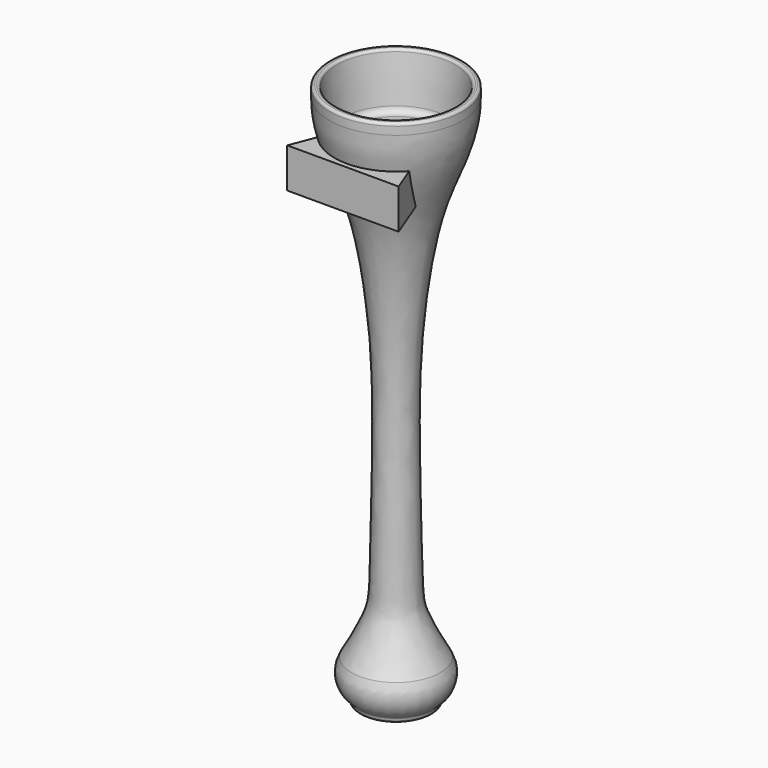
from build123d import *
from build123d import SkipClean  # not in build123d's __all__

# Parameters (mm, degrees)
F3_W     = 38.1
F3_H     = 19.05
F6_DEPTH = 19.05


with BuildPart() as f1:
    # F0 (on Front) → F1 (revolve)
    with BuildSketch(Plane.XZ):
        with BuildLine():
            Line((0, 215.9), (0, 34.925))
            Line((0, 34.925), (4.7625, 34.925))
            Line((4.7625, 34.925), (4.7625, 0))
            Line((4.7625, 0), (16.0301817854, 0))
            ThreePointArc((16.0301817854, 0), (16.8033088002, 0.2624412578), (17.2569075847, 0.9412998127))
            Line((17.2569075847, 0.9412998127), (17.5491598191, 2.032))
            ThreePointArc((17.5491598191, 2.032), (17.7163700396, 2.4035331582), (17.9926232895, 2.7029998297))
            ThreePointArc((17.9926232895, 2.7029998297), (22.6317424543, 10.3029935013), (21.1404360837, 19.0812242878))
            add(Edge.make_bspline(
                [(31.75, 255.27), (31.75, 245.2107101672), (26.5185945183, 228.7014550673), (15.9844015161, 205.2210464666), (8.947216643, 154.5246702551), (8.6661346378, 107.7502824908), (10.0068103161, 49.8637921648), (10.5640065806, 38.5089857021), (18.5789449872, 23.4888877699), (21.1404360837, 19.0812242878)],
                knots=[0, 0, 0, 0, 0.129505276, 0.2557549168, 0.4313220358, 0.6126472182, 0.7978183645, 0.8863622153, 1, 1, 1, 1], degree=3))
            Line((31.75, 255.27), (31.75, 259.08))
            ThreePointArc((31.75, 259.08), (31.3780256121, 259.9780256121), (30.48, 260.35))
            Line((30.48, 260.35), (29.698601086, 260.35))
            ThreePointArc((29.698601086, 260.35), (28.8570736248, 260.0311737654), (28.4380674734, 259.2347740661))
            Line((28.4380674734, 259.2347740661), (25.7986034696, 237.7380648347))
            ThreePointArc((25.7986034696, 237.7380648347), (24.7510880912, 235.7470655865), (22.6472694381, 234.95))
            Line((22.6472694381, 234.95), (3.175, 234.95))
            Line((3.175, 234.95), (3.175, 215.9))
            Line((3.175, 215.9), (0, 215.9))
        make_face()
    revolve(axis=Axis((0, 0, 125.4125), (0, 0, 1)))

    # F3 (on offset) → F4 (join, up to the next surface of F1)
    with BuildSketch(Plane.XZ.offset(31.75)):
        with Locations((0, 229.235)):
            Rectangle(F3_W, F3_H)
    extrude(until=Until.NEXT, dir=(0, 1, 0))

    # F5 (on face) → F6 (join, through all)
    with BuildSketch(Plane.XY.offset(238.76)):
        Polygon((19.05, -11.9982660867), (19.05, -31.75), (26.67, -31.75), align=None)
        Polygon((-19.05, -11.9982660867), (-26.67, -31.75), (-19.05, -31.75), align=None)
    extrude(amount=-F6_DEPTH)

    # F7 (on Front) → F8 (revolve, cut)
    with BuildSketch(Plane.XZ):
        with BuildLine():
            Line((25.7986034696, 237.7380648347), (28.9941972857, 263.7640879161))
            Line((28.9941972857, 263.7640879161), (0, 263.7158632278))
            Line((0, 263.7158632278), (0, 234.95))
            Line((0, 234.95), (22.6472694381, 234.95))
            ThreePointArc((22.6472694381, 234.95), (24.7510880912, 235.7470655865), (25.7986034696, 237.7380648347))
        make_face()
    with SkipClean():  # cleaning this boolean's faces spoils the solid; the shape is the same uncleaned
        revolve(axis=Axis((0, 0, 155.8669472579), (0, 0, 1)), mode=Mode.SUBTRACT)


solid = f1.part
